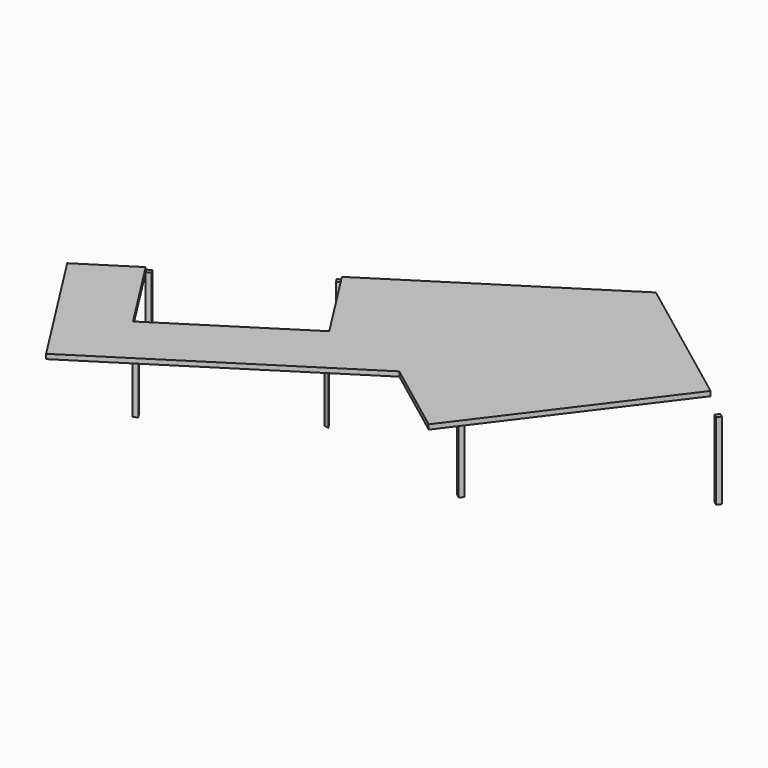
from build123d import *

# Parameters (mm, degrees)
F1_DEPTH = 152.4
F3_DEPTH = 2500


# Not quite as in the source:
# - a feature names something its author has since deleted; it is built from what else it names


with BuildPart() as f1:
    # F0 (on Top) → F1 (new body)
    with BuildSketch(Plane.XY):
        Polygon((-10792.6881330665, 5258.6957760002), (-11635.931151615, 4721.163254501), (-11098.3986301158, 3877.9202359526), (-10255.1556115673, 4415.4527574517), align=None)
        Polygon((-10255.1556115673, 4415.4527574517), (-11098.3986301158, 3877.9202359526), (-10560.8661086167, 3034.6772174041), (-9717.6230900682, 3572.2097389032), align=None)
        Polygon((-9949.445114518, 5796.2282974993), (-10792.6881330665, 5258.6957760002), (-10255.1556115673, 4415.4527574517), (-9411.9125930189, 4952.9852789509), align=None)
        Polygon((-9717.6230900682, 3572.2097389032), (-10560.8661086167, 3034.6772174041), (-10023.3335871175, 2191.4341988556), (-9180.090568569, 2728.9667203547), align=None)
        Polygon((-9411.9125930189, 4952.9852789509), (-10255.1556115673, 4415.4527574517), (-9717.6230900682, 3572.2097389032), (-8874.3800715197, 4109.7422604024), align=None)
        Polygon((-9180.090568569, 2728.9667203547), (-10023.3335871175, 2191.4341988556), (-9485.8010656184, 1348.1911803071), (-8642.5580470699, 1885.7237018062), align=None)
        Polygon((-8874.3800715197, 4109.7422604024), (-9717.6230900682, 3572.2097389032), (-9180.090568569, 2728.9667203547), (-8336.8475500206, 3266.4992418539), align=None)
        Polygon((-8642.5580470699, 1885.7237018062), (-9485.8010656184, 1348.1911803071), (-8948.2685441192, 504.9481617586), (-8105.0255255708, 1042.4806832577), align=None)
        Polygon((-8336.8475500206, 3266.4992418539), (-9180.090568569, 2728.9667203547), (-8642.5580470699, 1885.7237018062), (-7799.3150285214, 2423.2562233054), align=None)
        Polygon((-7799.3150285214, 2423.2562233054), (-8642.5580470699, 1885.7237018062), (-8105.0255255708, 1042.4806832577), (-7261.7825070223, 1580.0132047569), align=None)
        Polygon((-7493.6045314721, 3804.031763353), (-8336.8475500206, 3266.4992418539), (-7799.3150285214, 2423.2562233054), (-6956.0720099729, 2960.7887448045), align=None)
        Polygon((-6956.0720099729, 2960.7887448045), (-7799.3150285214, 2423.2562233054), (-7261.7825070223, 1580.0132047569), (-6418.5394884738, 2117.545726256), align=None)
        Polygon((-6650.3615129236, 4341.5642848522), (-7493.6045314721, 3804.031763353), (-6956.0720099729, 2960.7887448045), (-6112.8289914244, 3498.3212663037), align=None)
        Polygon((-6112.8289914244, 3498.3212663037), (-6956.0720099729, 2960.7887448045), (-6418.5394884738, 2117.545726256), (-5575.2964699253, 2655.0782477552), align=None)
        Polygon((-5807.1184943751, 4879.0968063513), (-6650.3615129236, 4341.5642848522), (-6112.8289914244, 3498.3212663037), (-5269.5859728759, 4035.8537878028), align=None)
        Polygon((-5269.5859728759, 4035.8537878028), (-6112.8289914244, 3498.3212663037), (-5575.2964699253, 2655.0782477552), (-4732.0534513768, 3192.6107692543), align=None)
        Polygon((-4963.8754758266, 5416.6293278505), (-5807.1184943751, 4879.0968063513), (-5269.5859728759, 4035.8537878028), (-4426.3429543275, 4573.386309302), align=None)
        Polygon((-4426.3429543275, 4573.386309302), (-5269.5859728759, 4035.8537878028), (-4732.0534513768, 3192.6107692543), (-3888.8104328283, 3730.1432907535), align=None)
        Polygon((-4120.6324572781, 5954.1618493496), (-4963.8754758266, 5416.6293278505), (-4426.3429543275, 4573.386309302), (-3583.099935779, 5110.9188308011), align=None)
        Polygon((-3583.099935779, 5110.9188308011), (-4426.3429543275, 4573.386309302), (-3888.8104328283, 3730.1432907535), (-3045.5674142798, 4267.6758122526), align=None)
        Polygon((-3277.3894387296, 6491.6943708488), (-4120.6324572781, 5954.1618493496), (-3583.099935779, 5110.9188308011), (-2739.8569172305, 5648.4513523003), align=None)
        Polygon((-4658.1649787773, 6797.4048678981), (-4120.6324572781, 5954.1618493496), (-3277.3894387296, 6491.6943708488), (-3814.9219602288, 7334.9373893972), align=None)
        Polygon((-2739.8569172305, 5648.4513523003), (-3583.099935779, 5110.9188308011), (-3045.5674142798, 4267.6758122526), (-2202.3243957313, 4805.2083337518), align=None)
        Polygon((-5195.6975002764, 7640.6478864466), (-4658.1649787773, 6797.4048678981), (-3814.9219602288, 7334.9373893972), (-4352.4544817279, 8178.1804079457), align=None)
        Polygon((-2434.1464201811, 7029.2268923479), (-3277.3894387296, 6491.6943708488), (-2739.8569172305, 5648.4513523003), (-1896.613898682, 6185.9838737994), align=None)
        Polygon((-3814.9219602288, 7334.9373893972), (-3277.3894387296, 6491.6943708488), (-2434.1464201811, 7029.2268923479), (-2971.6789416803, 7872.4699108964), align=None)
        Polygon((-1896.613898682, 6185.9838737994), (-2739.8569172305, 5648.4513523003), (-2202.3243957313, 4805.2083337518), (-1359.0813771828, 5342.7408552509), align=None)
        Polygon((-5733.2300217756, 8483.8909049951), (-5195.6975002764, 7640.6478864466), (-4352.4544817279, 8178.1804079457), (-4889.9870032271, 9021.4234264942), align=None)
        Polygon((-4352.4544817279, 8178.1804079457), (-3814.9219602288, 7334.9373893972), (-2971.6789416803, 7872.4699108964), (-3509.2114631794, 8715.7129294449), align=None)
        Polygon((-1857.8527060458, 7396.590281631), (-2434.1464201811, 7029.2268923479), (-1896.613898682, 6185.9838737994), (-1608.4670416143, 6369.6655684409), align=None)
        Polygon((-2971.6789416803, 7872.4699108964), (-2434.1464201811, 7029.2268923479), (-1857.8527060458, 7396.590281631), (-2107.2383704773, 8423.514994821), align=None)
        Polygon((-1608.4670416143, 6369.6655684409), (-1896.613898682, 6185.9838737994), (-1359.0813771828, 5342.7408552509), align=None)
        Polygon((-4889.9870032271, 9021.4234264942), (-4352.4544817279, 8178.1804079457), (-3509.2114631794, 8715.7129294449), (-4046.7439846786, 9558.9559479934), align=None)
        Polygon((-3509.2114631794, 8715.7129294449), (-2971.6789416803, 7872.4699108964), (-2107.2383704773, 8423.514994821), (-2356.6240349088, 9450.439708011), align=None)
        Polygon((-2107.2383704773, 8423.514994821), (-1857.8527060458, 7396.590281631), (-1084.9575905035, 7889.2789267465), (-947.8956971639, 9162.5479624944), align=None)
        Polygon((-1084.9575905035, 7889.2789267465), (-1857.8527060458, 7396.590281631), (-1608.4670416143, 6369.6655684409), (-1222.0194838432, 6616.0098909987), align=None)
        Polygon((-697.9368235911, 6221.881275921), (-1359.0813771828, 5342.7408552509), (-559.8628129373, 4741.7003519857), (101.2817406544, 5620.8407726558), align=None)
        Polygon((-851.5780562803, 6337.4248930854), (-1359.0813771828, 5342.7408552509), (-697.9368235911, 6221.881275921), align=None)
        Polygon((-1608.4670416143, 6369.6655684409), (-1359.0813771828, 5342.7408552509), (-1222.0194838432, 6616.0098909987), align=None)
        Polygon((-1222.0194838432, 6616.0098909987), (-1359.0813771828, 5342.7408552509), (-1005.2192889696, 6452.9685102497), align=None)
        Polygon((-1005.2192889696, 6452.9685102497), (-1359.0813771828, 5342.7408552509), (-851.5780562803, 6337.4248930854), align=None)
        Polygon((-4046.7439846786, 9558.9559479934), (-3509.2114631794, 8715.7129294449), (-2356.6240349088, 9450.439708011), (-2606.0096993403, 10477.364421201), align=None)
        Polygon((-2356.6240349088, 9450.439708011), (-2107.2383704773, 8423.514994821), (-947.8956971639, 9162.5479624944), (-810.8338038243, 10435.8169982422), align=None)
        Polygon((-947.8956971639, 9162.5479624944), (-1084.9575905035, 7889.2789267465), (-651.3572007564, 7563.1961652486), (-297.4951125431, 8673.4238202474), align=None)
        Polygon((-651.3572007564, 7563.1961652486), (-1084.9575905035, 7889.2789267465), (-1222.0194838432, 6616.0098909987), (-1005.2192889696, 6452.9685102497), align=None)
        Polygon((101.2817406544, 5620.8407726558), (-559.8628129373, 4741.7003519857), (239.3557513082, 4140.6598487205), (900.5003049, 5019.8002693906), align=None)
        Polygon((-851.5780562803, 6337.4248930854), (-697.9368235911, 6221.881275921), (-36.7922699994, 7101.0216965911), (-344.0747353779, 7332.1089309198), align=None)
        Polygon((-36.7922699994, 7101.0216965911), (-697.9368235911, 6221.881275921), (101.2817406544, 5620.8407726558), (762.4262942462, 6499.9811933259), align=None)
        Polygon((-651.3572007564, 7563.1961652486), (-1005.2192889696, 6452.9685102497), (-851.5780562803, 6337.4248930854), (-344.0747353779, 7332.1089309198), align=None)
        Polygon((-2606.0096993403, 10477.364421201), (-2356.6240349088, 9450.439708011), (-810.8338038243, 10435.8169982422), (-673.7719104846, 11709.08603399), align=None)
        Polygon((-810.8338038243, 10435.8169982422), (-947.8956971639, 9162.5479624944), (-297.4951125431, 8673.4238202474), (56.3669756701, 9783.6514752462), align=None)
        Polygon((-297.4951125431, 8673.4238202474), (-651.3572007564, 7563.1961652486), (-344.0747353779, 7332.1089309198), (163.4285855246, 8326.7929687543), align=None)
        Polygon((900.5003049, 5019.8002693906), (239.3557513082, 4140.6598487205), (1038.5743155538, 3539.6193454553), (1699.7188691455, 4418.7597661254), align=None)
        Polygon((762.4262942462, 6499.9811933259), (101.2817406544, 5620.8407726558), (900.5003049, 5019.8002693906), (1561.6448584917, 5898.9406900607), align=None)
        Polygon((-344.0747353779, 7332.1089309198), (-36.7922699994, 7101.0216965911), (624.3522835924, 7980.1621172612), (163.4285855246, 8326.7929687543), align=None)
        Polygon((624.3522835924, 7980.1621172612), (-36.7922699994, 7101.0216965911), (762.4262942462, 6499.9811933259), (1423.5708478379, 7379.121613996), align=None)
        Polygon((-673.7719104846, 11709.08603399), (-810.8338038243, 10435.8169982422), (56.3669756701, 9783.6514752462), (410.2290638833, 10893.879130245), align=None)
        Polygon((56.3669756701, 9783.6514752462), (-297.4951125431, 8673.4238202474), (163.4285855246, 8326.7929687543), (670.9319064271, 9321.4770065887), align=None)
        Polygon((1561.6448584917, 5898.9406900607), (900.5003049, 5019.8002693906), (1699.7188691455, 4418.7597661254), (2360.8634227372, 5297.9001867954), align=None)
        Polygon((1423.5708478379, 7379.121613996), (762.4262942462, 6499.9811933259), (1561.6448584917, 5898.9406900607), (2222.7894120835, 6778.0811107308), align=None)
        Polygon((163.4285855246, 8326.7929687543), (624.3522835924, 7980.1621172612), (1285.4968371841, 8859.3025379313), (670.9319064271, 9321.4770065887), align=None)
        Polygon((1285.4968371841, 8859.3025379313), (624.3522835924, 7980.1621172612), (1423.5708478379, 7379.121613996), (2084.7154014297, 8258.2620346661), align=None)
        Polygon((226.7158552526, 12283.1097123941), (-673.7719104846, 11709.08603399), (410.2290638833, 10893.879130245), (731.9218713499, 11903.1769984257), align=None)
        Polygon((410.2290638833, 10893.879130245), (56.3669756701, 9783.6514752462), (670.9319064271, 9321.4770065887), (1178.4352273296, 10316.1610444232), align=None)
        Polygon((2222.7894120835, 6778.0811107308), (1561.6448584917, 5898.9406900607), (2360.8634227372, 5297.9001867954), (3022.007976329, 6177.0406074655), align=None)
        Polygon((2084.7154014297, 8258.2620346661), (1423.5708478379, 7379.121613996), (2222.7894120835, 6778.0811107307), (2883.9339656752, 7657.2215314008), align=None)
        Polygon((670.9319064271, 9321.4770065887), (1285.4968371841, 8859.3025379313), (1946.6413907759, 9738.4429586014), (1178.4352273296, 10316.1610444232), align=None)
        Polygon((1946.6413907759, 9738.4429586014), (1285.4968371841, 8859.3025379313), (2084.7154014297, 8258.2620346661), (2745.8599550214, 9137.4024553361), align=None)
        Polygon((1012.7141266124, 12784.1510769883), (226.7158552526, 12283.1097123941), (731.9218713499, 11903.1769984257), align=None)
        Polygon((731.9218713499, 11903.1769984257), (410.2290638833, 10893.879130245), (1178.4352273296, 10316.1610444232), (1639.8018826955, 11220.4192606363), align=None)
        Polygon((2883.9339656752, 7657.2215314008), (2222.7894120835, 6778.0811107308), (3022.007976329, 6177.0406074655), (3683.1525299207, 7056.1810281356), align=None)
        Polygon((2745.8599550214, 9137.4024553361), (2084.7154014297, 8258.2620346661), (2883.9339656752, 7657.2215314008), (3545.0785192669, 8536.3619520709), align=None)
        Polygon((1178.4352273296, 10316.1610444232), (1946.6413907759, 9738.4429586014), (2547.6818940411, 10537.6615228469), (1639.8018826955, 11220.4192606363), align=None)
        Polygon((2547.6818940411, 10537.6615228469), (1946.6413907759, 9738.4429586014), (2745.8599550214, 9137.4024553361), (3346.9004582866, 9936.6210195817), align=None)
        Polygon((2042.5096232985, 12009.7086012022), (1012.7141266124, 12784.1510769883), (731.9218713499, 11903.1769984257), (1639.8018826955, 11220.4192606363), align=None)
        Polygon((3545.0785192669, 8536.3619520709), (2883.9339656752, 7657.2215314008), (3683.1525299207, 7056.1810281356), (4344.2970835125, 7935.3214488057), align=None)
        Polygon((3346.9004582866, 9936.6210195817), (2745.8599550214, 9137.4024553361), (3545.0785192669, 8536.3619520709), (4146.1190225322, 9335.5805163165), align=None)
        Polygon((1639.8018826955, 11220.4192606363), (2547.6818940411, 10537.6615228469), (3072.3051199846, 11235.2661254162), (2042.5096232985, 12009.7086012022), align=None)
        Polygon((3072.3051199846, 11235.2661254162), (2547.6818940411, 10537.6615228469), (3346.9004582866, 9936.6210195817), (3871.5236842301, 10634.225622151), align=None)
        Polygon((4146.1190225322, 9335.5805163165), (3545.0785192669, 8536.3619520709), (4344.2970835125, 7935.3214488057), (4945.3375867777, 8734.5400130512), align=None)
        Polygon((3871.5236842301, 10634.225622151), (3346.9004582866, 9936.6210195817), (4146.1190225322, 9335.5805163165), (4670.7422484756, 10033.1851188858), align=None)
        Polygon((4670.7422484756, 10033.1851188858), (4146.1190225322, 9335.5805163165), (4945.3375867777, 8734.5400130512), (5469.9608127212, 9432.1446156205), align=None)
    extrude(amount=-F1_DEPTH)

    # F2 (on face) → F3, piece 5 (join)
    with BuildSketch(Plane(origin=(0, 0, -152.4), x_dir=(1, 0, 0), z_dir=(0, 0, -1))):
        Polygon((-8254.9275937441, -3137.9890058271), (-8336.8475500206, -3266.4992418539), (-8208.3373139938, -3348.4191981303), (-8126.4173577173, -3219.9089621036), align=None)
        Polygon((-4153.5767600269, -5805.3652334056), (-4120.6324572781, -5954.1618493496), (-4004.7801440829, -5772.4209306568), align=None)
        Polygon((840.3962545735, -4939.878412966), (931.9948272711, -5061.679322157), (1053.7957364621, -4970.0807494594), (962.1971637645, -4848.2798402684), align=None)
    extrude(amount=F3_DEPTH)


with BuildPart() as f3:
    # F2 (on face) → F3 (new body)
    with BuildSketch(Plane(origin=(0, 0, -152.4), x_dir=(1, 0, 0), z_dir=(0, 0, -1))):
        Polygon((-9820.9348784912, -5878.1482537758), (-9949.445114518, -5796.2282974994), (-10031.3650707945, -5924.7385335262), (-9902.8548347677, -6006.6584898026), align=None)
    extrude(amount=F3_DEPTH)


with BuildPart() as f3b:
    # F2 (on face) → F3, piece 2 (new body)
    with BuildSketch(Plane(origin=(0, 0, -152.4), x_dir=(1, 0, 0), z_dir=(0, 0, -1))):
        Polygon((-5815.149978052, -8612.4011410219), (-5733.2300217756, -8483.8909049951), (-5861.7402578024, -8401.9709487186), (-5943.6602140788, -8530.4811847454), align=None)
    extrude(amount=F3_DEPTH)


with BuildPart() as f3c:
    # F2 (on face) → F3, piece 3 (new body)
    with BuildSketch(Plane(origin=(0, 0, -152.4), x_dir=(1, 0, 0), z_dir=(0, 0, -1))):
        Polygon((930.7941703359, -12912.661313015), (1012.7141266124, -12784.1510769883), (884.2038905856, -12702.2311207118), (802.2839343091, -12830.7413567386), align=None)
    extrude(amount=F3_DEPTH)


with BuildPart() as f3d:
    # F2 (on face) → F3, piece 4 (new body)
    with BuildSketch(Plane(origin=(0, 0, -152.4), x_dir=(1, 0, 0), z_dir=(0, 0, -1))):
        Polygon((6177.5808042691, -8709.3032031643), (6269.1793769667, -8831.1041123553), (6390.9802861577, -8739.5055396577), (6299.3817134601, -8617.7046304667), align=None)
    extrude(amount=F3_DEPTH)


with BuildPart() as f3e:
    # F2 (on face) → F3, piece 6 (new body)
    with BuildSketch(Plane(origin=(0, 0, -152.4), x_dir=(1, 0, 0), z_dir=(0, 0, -1))):
        Polygon((-2360.2579475816, -10634.0209909917), (-2488.7681836084, -10552.1010347152), (-2570.6881398848, -10680.611270742), (-2442.1779038581, -10762.5312270185), align=None)
    extrude(amount=F3_DEPTH)


solid = Compound([f1.part, f3.part, f3b.part, f3c.part, f3d.part, f3e.part])
